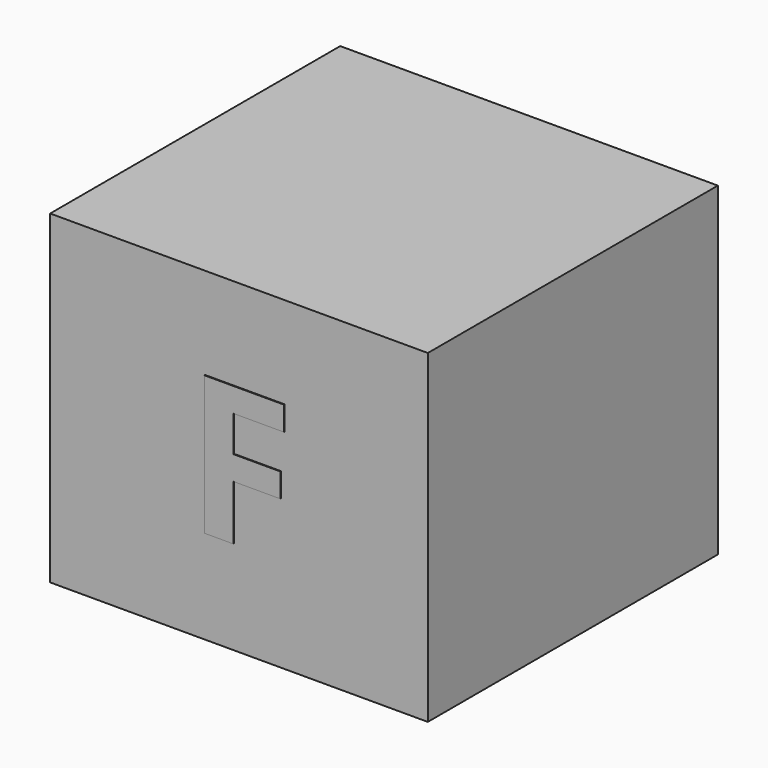
from build123d import *

# Parameters (mm, degrees)
F0_W         = 500
F0_H         = 480
F1_DEPTH     = 430
F2_TEXT_SIZE = 257.8243199322
F3_DEPTH     = 1


# Not quite as in the source:
# - Text() gives the source's letters only with a copy of the font that has no kerning and outlines rounded to 1/6400 em; it was checked with that copy


with BuildPart() as f1:
    # F0 (on Top) → F1 (new body)
    with BuildSketch(Plane.XY):
        Rectangle(F0_W, F0_H)
    extrude(amount=F1_DEPTH)

    # F2 (on face) → F3 (join)
    with BuildSketch(Plane.XZ.offset(240)):
        with Locations((-68.2306746021, 124.4359463453)):
            Text('F', F2_TEXT_SIZE, font='Open Sans', font_style=FontStyle.BOLD, text_align=(TextAlign.LEFT, TextAlign.BOTTOM))
    extrude(amount=F3_DEPTH)


solid = f1.part
